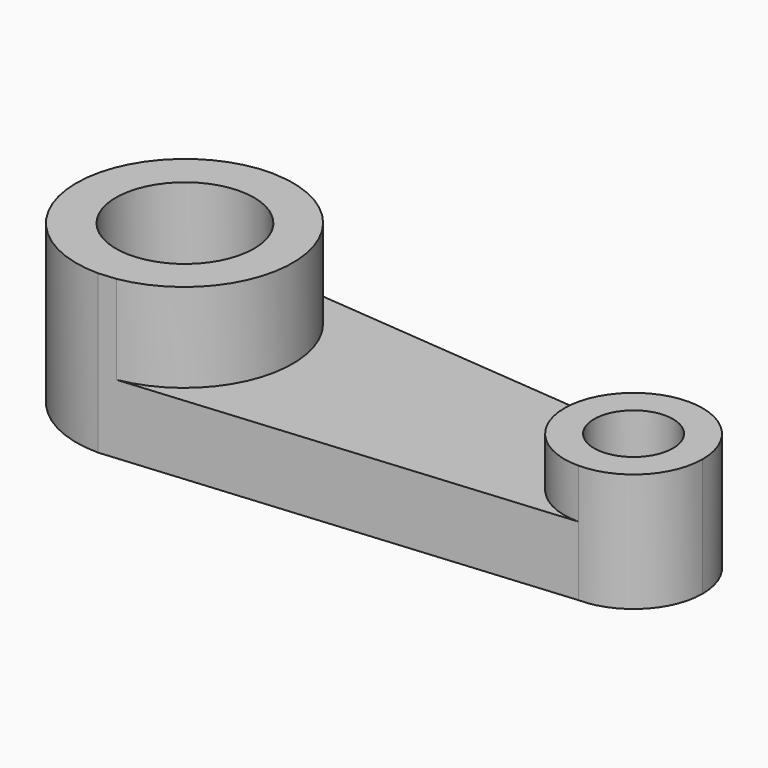
from build123d import *

# Parameters (mm, degrees)
F0_W      = 177.8
F0_H      = 50.8
F1_DEPTH  = 69.85
F3_DEPTH  = 50.8
F2_R      = 22.225
F4_DEPTH  = 50.8
F5_DEPTH  = 50.8
F7_DEPTH  = 50.8
F6_R      = 12.7
F8_DEPTH  = 50.8
F10_DEPTH = 50.8
F12_DEPTH = 28.575
F13_R     = 22.225
F14_DEPTH = 12.7


# Not quite as in the source:
# - ends of sketch curves that miss each other by under 0.0002 mm in the source are joined


with BuildPart() as f1:
    # F0 (on Front) → F1 (new body)
    with BuildSketch(Plane.XZ):
        with Locations((88.9, 25.4)):
            Rectangle(F0_W, F0_H)
    extrude(amount=F1_DEPTH)

    # F2 (on face) → F3 (cut, through all)
    with BuildSketch(Plane.XY.offset(50.8)):
        with BuildLine():
            Line((0, -69.85), (34.925, -69.85))
            ThreePointArc((34.925, -69.85), (10.2292956671, -59.6207043329), (0, -34.925))
            Line((0, -34.925), (0, -69.85))
        make_face()
        with BuildLine():
            ThreePointArc((0, -34.925), (10.2292957417, -10.2292955924), (34.9250002112, 0))
            Line((34.9250002112, 0), (0, 0))
            Line((0, 0), (0, -34.925))
        make_face()
    extrude(amount=-F3_DEPTH, mode=Mode.SUBTRACT)

    # F2 (on face) → F4 (cut, through all)
    with BuildSketch(Plane.XY.offset(50.8)):
        with Locations((34.925, -34.925)):
            Circle(F2_R)
    extrude(amount=-F4_DEPTH, mode=Mode.SUBTRACT)

    # F5 (add): a face of the model
    f5_faces = [f1.faces().sort_by_distance(p)[0] for p in [
        (177.8, -34.925, 25.4),
    ]]
    extrude(f5_faces, amount=F5_DEPTH)

    # F6 (on face) → F7 (cut, through all)
    with BuildSketch(Plane.XY.offset(50.8)):
        with BuildLine():
            Line((228.6, 0), (34.9250002112, 0))
            Line((34.9250002112, 0), (180.975, -10.3535739202))
            ThreePointArc((180.975, -10.3535739202), (203.8662068568, -34.925), (180.975, -59.4964260798))
            Line((180.975, -59.4964260798), (34.925, -69.85))
            Line((34.925, -69.85), (228.6, -69.85))
            Line((228.6, -69.85), (228.6, 0))
        make_face()
    extrude(amount=-F7_DEPTH, mode=Mode.SUBTRACT)

    # F6 (on face) → F8 (cut, through all)
    with BuildSketch(Plane.XY.offset(50.8)):
        with Locations((179.2331165612, -34.925)):
            Circle(F6_R)
    extrude(amount=-F8_DEPTH, mode=Mode.SUBTRACT)

    # F9 (on face) → F10 (cut, through all)
    with BuildSketch(Plane.XY.offset(50.8)):
        with BuildLine():
            ThreePointArc((179.2331165612, -12.7), (194.948564773, -19.2095517881), (201.4581165612, -34.925))
            ThreePointArc((201.4581165612, -34.925), (194.948564773, -50.6404482119), (179.2331165612, -57.15))
            Line((179.2331165612, -57.15), (34.925, -69.85))
            Line((34.925, -69.85), (180.975, -59.4964260798))
            ThreePointArc((180.975, -59.4964260798), (203.8662068568, -34.925), (180.975, -10.3535739202))
            Line((180.975, -10.3535739202), (34.9250002112, 0))
            Line((34.9250002112, 0), (179.2331165612, -12.7))
        make_face()
    extrude(amount=-F10_DEPTH, mode=Mode.SUBTRACT)

    # F11 (on face) → F12 (cut)
    with BuildSketch(Plane.XY.offset(50.8)):
        with BuildLine():
            ThreePointArc((40.4881105931, -0.4895878599), (69.5805320507, -34.9249998886), (40.4881108127, -69.3604121029))
            Line((40.4881108127, -69.3604121029), (179.2331165612, -57.15))
            ThreePointArc((179.2331165612, -57.15), (157.0081165612, -34.925), (179.2331165612, -12.7))
            Line((179.2331165612, -12.7), (40.4881105931, -0.4895878599))
        make_face()
    extrude(amount=-F12_DEPTH, mode=Mode.SUBTRACT)

    # F13 (on face) → F14 (cut)
    with BuildSketch(Plane.XY.offset(50.8)):
        with Locations((179.2331165612, -34.925)):
            Circle(F13_R)
    extrude(amount=-F14_DEPTH, mode=Mode.SUBTRACT)


solid = f1.part
